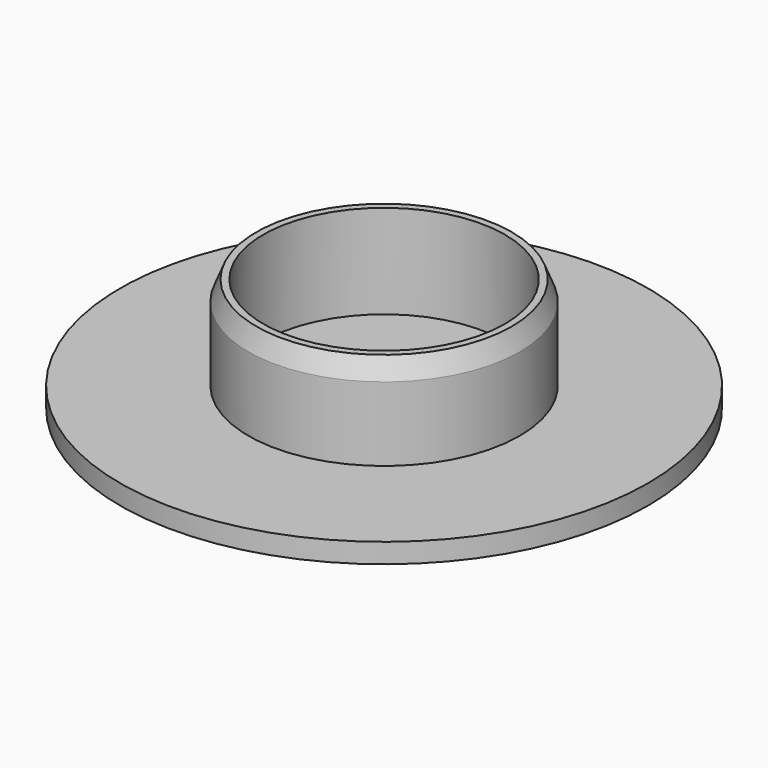
from build123d import *

# Parameters (mm, degrees)
F0_R     = 26.75
F1_DEPTH = 2
F2_R     = 13.75
F2_R_2   = 12.25
F3_DEPTH = 9.5
F4_SIZE2 = 2
F4_SIZE  = 0.8
F5_R     = 5.5
F6_DEPTH = 25


# Not quite as in the source:
# - a feature of the source that left no trace in its solid (it failed there, or was rolled back) is left out


with BuildPart() as f1:
    # F0 (on Top) → F1 (new body)
    with BuildSketch(Plane.XY):
        Circle(F0_R)
    extrude(amount=F1_DEPTH)

    # F2 (on face) → F3 (join)
    with BuildSketch(Plane.XY.offset(2)):
        Circle(F2_R)
        Circle(F2_R_2, mode=Mode.SUBTRACT)
    extrude(amount=F3_DEPTH)

    # F4
    f4_edges = [f1.edges().sort_by_distance(p)[0] for p in [
        (-13.75, 0, 11.5),
    ]]
    f4_side = f1.faces().sort_by_distance((-13.361091, 0, 11.5))[0]
    chamfer(f4_edges, length=F4_SIZE, length2=F4_SIZE2, reference=f4_side)

    # F5 (on face) → F6 (cut)
    with BuildSketch(Plane.XY.offset(2)):
        Circle(F5_R)
    extrude(amount=-F6_DEPTH, mode=Mode.SUBTRACT)


solid = f1.part
